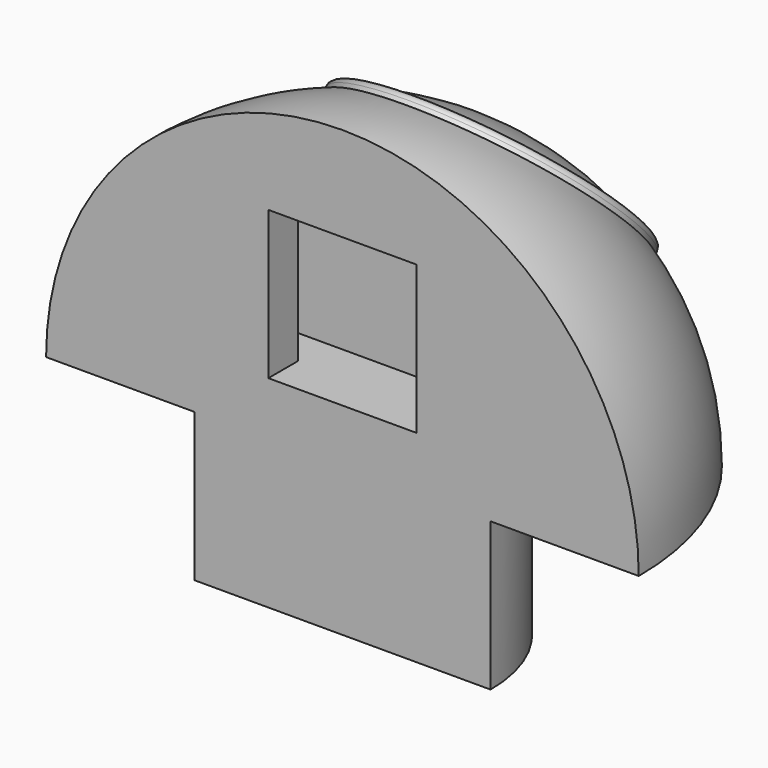
from build123d import *

# Parameters (mm, degrees)
F1_ANGLE  = 180
F12_R     = 6.1952157487
F12_R_2   = 5.6872157487
F13_DEPTH = 2.54
F18_W     = 6.35
F18_H     = 6.35
F19_DEPTH = 3.175
F21_W     = 1.5875
F21_H     = 6.35
F22_DEPTH = 1.5875
F20_W     = 1.5875
F20_H     = 6.35
F23_DEPTH = 1.5875


# Not quite as in the source:
# - a fillet or chamfer that OpenCascade refuses, or shapes differently, is made with other operations: its cross-section is extruded or revolved along the edge and cut away or added


with BuildPart() as f1:
    # F0 (on Front) → F1 (revolve)
    with BuildSketch(Plane.XZ):
        with BuildLine():
            Line((6.35, 0), (12.7, 0))
            ThreePointArc((12.7, 0), (8.9802561211, 8.9802561211), (0, 12.7))
            Line((0, 12.7), (0, 0))
            Line((0, 0), (0, -6.35))
            Line((0, -6.35), (6.35, -6.35))
            Line((6.35, -6.35), (6.35, 0))
        make_face()
    revolve(axis=Axis((0, 0, 3.175), (0, 0, 1)), revolution_arc=F1_ANGLE)

    # F4 (on offset) → F5 (revolve)
    with BuildSketch(Plane.XZ.offset(-5.334)):
        with BuildLine():
            ThreePointArc((2.4398909882, -1.3480047928), (1.5384289576, -2.5219143718), (2.4398909882, -3.6958239507))
            Line((2.4398909882, -3.6958239507), (2.4398909882, -1.3480047928))
        make_face()
    revolve(axis=Axis((2.4398909882, 5.334, -2.5219143718), (0, 0, -1)))

    # F6 (on offset) → F7 (revolve)
    with BuildSketch(Plane.XZ.offset(-5.334)):
        with BuildLine():
            ThreePointArc((-2.4398909882, -3.6958239507), (-1.5384289576, -2.5219143718), (-2.4398909882, -1.3480047928))
            Line((-2.4398909882, -1.3480047928), (-2.4398909882, -3.6958239507))
        make_face()
    revolve(axis=Axis((-2.4398909882, 5.334, -2.5219143718), (0, 0, -1)))

    # F12 (on 3pt) → F13 (join)
    with BuildSketch(Plane(origin=(0, 6.35, 6.35), x_dir=(1, 0, 0), z_dir=(0, 0.7071067812, 0.7071067812))):
        Circle(F12_R)
        Circle(F12_R_2, mode=Mode.SUBTRACT)
    extrude(amount=F13_DEPTH)

    # F14: fillet of radius 0.254 on 2 edges, made by hand

    # F14_s1 → F14_t2 (revolve, cut)
    with BuildSketch(Plane(origin=(0, 0, 0), x_dir=(1, 0, 0), z_dir=(0, -0.7071067812, 0.7071067812))):
        with BuildLine():
            ThreePointArc((6.1952157487, 11.2662561211), (6.1208208712, 11.4458612435), (5.9412157487, 11.5202561211))
            Line((5.9412157487, 11.5202561211), (6.1952157487, 11.5202561211))
            Line((6.1952157487, 11.5202561211), (6.1952157487, 11.2662561211))
        make_face()
    revolve(axis=Axis((0, 8.1460512242, 8.1460512242), (0, 0.7071067812, 0.7071067812)), mode=Mode.SUBTRACT)

    # F14_s3 → F14_t4 (revolve, cut)
    with BuildSketch(Plane(origin=(0, 0, 0), x_dir=(1, 0, 0), z_dir=(0, -0.7071067812, 0.7071067812))):
        with BuildLine():
            ThreePointArc((5.9250512041, 11.5202561211), (5.7803649537, 11.4750188787), (5.6872157662, 11.3554206011))
            Line((5.6872157662, 11.3554206011), (5.6872157487, 11.5202561211))
            Line((5.6872157487, 11.5202561211), (5.9250512041, 11.5202561211))
        make_face()
    revolve(axis=Axis((0, 8.1460512242, 8.1460512242), (0, 0.7071067812, 0.7071067812)), mode=Mode.SUBTRACT)

    # F18 (on face) → F19 (cut)
    with BuildSketch(Plane.XZ):
        with Locations((0, 5.478449179)):
            Rectangle(F18_W, F18_H)
    extrude(amount=-F19_DEPTH, mode=Mode.SUBTRACT)

    # F21 (on face) → F22 (cut)
    with BuildSketch(Plane.YZ.offset(-3.175)):
        with Locations((2.38125, 5.478449179)):
            Rectangle(F21_W, F21_H)
    extrude(amount=-F22_DEPTH, mode=Mode.SUBTRACT)

    # F20 (on face) → F23 (cut)
    with BuildSketch(Plane(origin=(3.175, 0, 0), x_dir=(0, -1, 0), z_dir=(-1, 0, 0))):
        with Locations((-2.38125, 5.478449179)):
            Rectangle(F20_W, F20_H)
    extrude(amount=-F23_DEPTH, mode=Mode.SUBTRACT)


solid = f1.part
